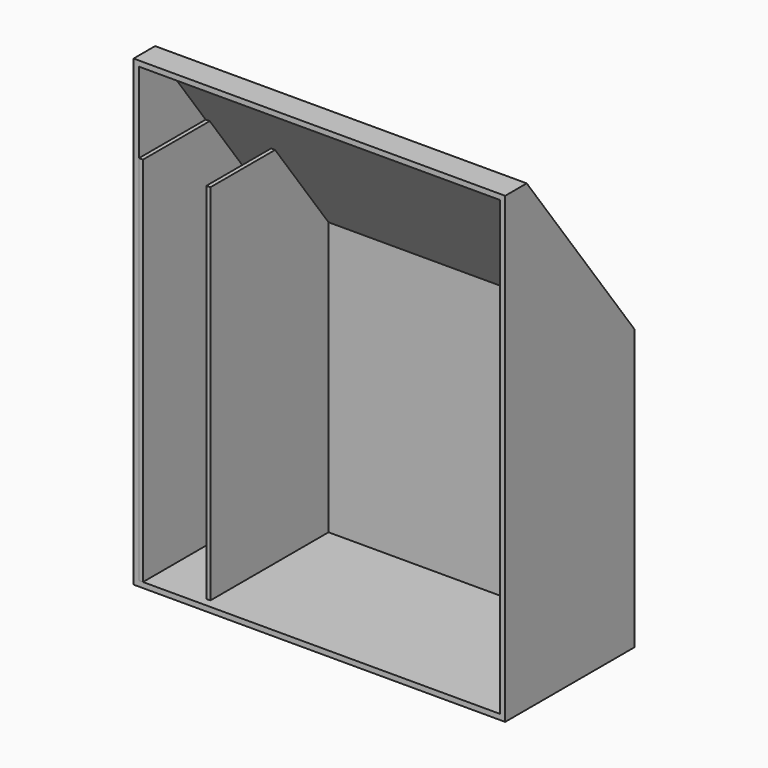
from build123d import *

# Parameters (mm, degrees)
F0_W     = 1752.6
F0_H     = 2184.4
F1_DEPTH = 762
F2_SIZE2 = 635
F2_SIZE  = 863.6
F3_T     = -25.4
F5_DEPTH = 19.05
F8_DEPTH = 19.05


with BuildPart() as f1:
    # F0 (on Front) → F1 (new body)
    with BuildSketch(Plane.XZ):
        with Locations((-110.9929393764, 27.8082511663)):
            Rectangle(F0_W, F0_H)
    extrude(amount=-F1_DEPTH)

    # F2
    f2_edges = [f1.edges().sort_by_distance(p)[0] for p in [
        (-110.992939, 762, 1120.008251),
    ]]
    f2_side = f1.faces().sort_by_distance((-110.992939, 762, 27.808251))[0]
    chamfer(f2_edges, length=F2_SIZE, length2=F2_SIZE2, reference=f2_side)

    # F3
    f3_openings = [f1.faces().sort_by_distance(p)[0] for p in [
        (-110.992939, 0, 27.808251),
    ]]
    offset(amount=F3_T, openings=f3_openings)


with BuildPart() as f5:
    # F4 (on face) → F5 (new body)
    with BuildSketch(Plane.YZ.offset(-961.8929393764)):
        Polygon((736.6, -1038.9917488337), (736.6, 248.0751251433), (393.5104036319, 714.6769762039), (0, 714.6769762039), (0, -1038.9917488337), align=None)
    extrude(amount=F5_DEPTH)


with BuildPart() as f8:
    # F7 (on offset) → F8 (new body)
    with BuildSketch(Plane.YZ.offset(-676.1429393764)):
        Polygon((776.6470954039, -1077.1855942721), (776.6470954039, 209.8812797048), (433.5574990358, 676.4831307655), (40.0470954039, 676.4831307655), (40.0470954039, -1077.1855942721), align=None)
    extrude(amount=F8_DEPTH)


solid = Compound([f1.part, f5.part, f8.part])
